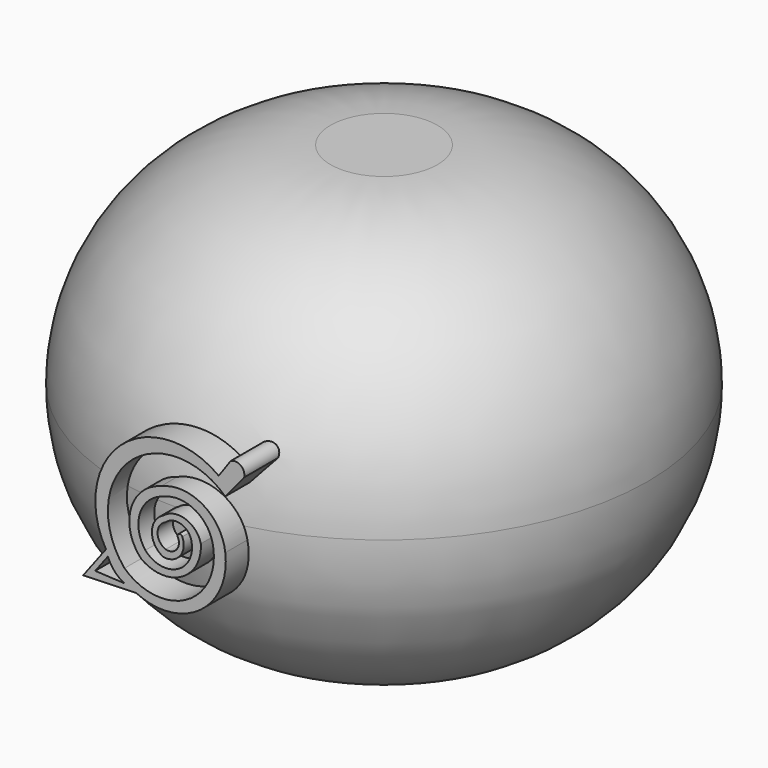
from build123d import *

# Parameters (mm, degrees)
F0_R     = 15.9252412
F1_DEPTH = 25.4
F2_R     = 12.69999
F5_DEPTH = 3.81


# Not quite as in the source:
# - a fillet or chamfer is up to 0.001 mm smaller than in the source, because OpenCascade refuses the exact size


with BuildPart() as f1:
    # F0 (on Top) → F1 (new body)
    with BuildSketch(Plane.XY):
        with Locations((-33.0793492307, 17.5561513754)):
            Circle(F0_R)
    extrude(amount=F1_DEPTH)

    # F2 (radius 12.7 in the source; OpenCascade refuses exactly that, so slightly less here)
    f2_edges = [f1.edges().sort_by_distance(p)[0] for p in [
        (-49.00459, 17.556151, 25.4),
        (-49.00459, 17.556151, 0),
    ]]
    fillet(f2_edges, radius=F2_R)

    # F4 (on offset) → F5 (join)
    with BuildSketch(Plane.XZ.offset(-4.318)):
        with BuildLine():
            Line((-29.0207639337, 14.9749675766), (-27.8811603785, 16.3556560874))
            ThreePointArc((-27.8811603785, 16.3556560874), (-28.0885315249, 16.9271168776), (-28.695197776, 16.9661846012))
            Line((-28.695197776, 16.9661846012), (-29.4164977968, 15.9463118762))
            ThreePointArc((-29.4164977968, 15.9463118762), (-35.315728181, 15.6618586245), (-36.2196562996, 9.8253573836))
            ThreePointArc((-36.2196562996, 9.8253573836), (-36.219121003, 9.824445743), (-36.2185855, 9.8235342236))
            Line((-36.2185855, 9.8235342236), (-37.5962145627, 8.0000562593))
            Line((-37.5962145627, 8.0000562593), (-34.392606223, 8.0947948317))
            ThreePointArc((-34.392606223, 8.0947948317), (-34.3897808352, 8.0934481012), (-34.3869543323, 8.0921037126))
            ThreePointArc((-34.3869543323, 8.0921037126), (-30.5469478577, 8.4474204279), (-29.0207639337, 11.9889825583))
            ThreePointArc((-29.0207639337, 11.9889825583), (-30.3891986708, 14.106652787), (-32.9061411321, 14.2554529011))
            ThreePointArc((-32.9061411321, 14.2554529011), (-34.717169495, 12.4733526926), (-34.0933389962, 10.0103178993))
            ThreePointArc((-34.0933389962, 10.0103178993), (-31.6624363369, 9.8503464108), (-30.4957684129, 11.9889825583))
            ThreePointArc((-30.4957684129, 11.9889825583), (-31.4214059538, 12.9964876797), (-32.7661586101, 12.7444723621))
            ThreePointArc((-32.7661586101, 12.7444723621), (-33.4490909653, 11.6472132504), (-32.7661586101, 10.5499541387))
            ThreePointArc((-32.7661586101, 10.5499541387), (-31.7571819842, 10.9231691425), (-31.6110141575, 11.9889825583))
            ThreePointArc((-31.6110141575, 11.9889825583), (-31.7935886004, 12.08811911), (-31.8988275295, 11.9089927555))
            ThreePointArc((-31.8988275295, 11.9089927555), (-31.9495376202, 11.212409195), (-32.6134748757, 10.9956432134))
            ThreePointArc((-32.6134748757, 10.9956432134), (-33.1081520423, 11.7169185542), (-32.6134748757, 12.4381938949))
            ThreePointArc((-32.6134748757, 12.4381938949), (-31.714287938, 12.6534772255), (-31.0713797808, 11.9889825583))
            ThreePointArc((-31.0713797808, 11.9889825583), (-31.8928919194, 10.1846295294), (-33.841509372, 10.5499541387))
            ThreePointArc((-33.841509372, 10.5499541387), (-34.1573684854, 12.4434120609), (-32.7527012902, 13.7517927215))
            ThreePointArc((-32.7527012902, 13.7517927215), (-30.7985222002, 13.6359080863), (-29.7402776778, 11.9889825583))
            ThreePointArc((-29.7402776778, 11.9889825583), (-31.4290089637, 8.6919853613), (-35.1006612182, 9.182875976))
            ThreePointArc((-35.1006612182, 9.182875976), (-34.7993943786, 14.9536870948), (-29.0207639337, 14.9749675766))
        make_face()
        with BuildLine():
            Line((-36.8709181573, 8.4690021479), (-36.0997095704, 9.489800781))
            ThreePointArc((-36.0997095704, 9.489800781), (-35.713386033, 8.8381304316), (-35.107601434, 8.383218199))
            Line((-35.107601434, 8.383218199), (-36.8709181573, 8.4690021479))
        make_face(mode=Mode.SUBTRACT)
    extrude(amount=F5_DEPTH)


solid = f1.part
